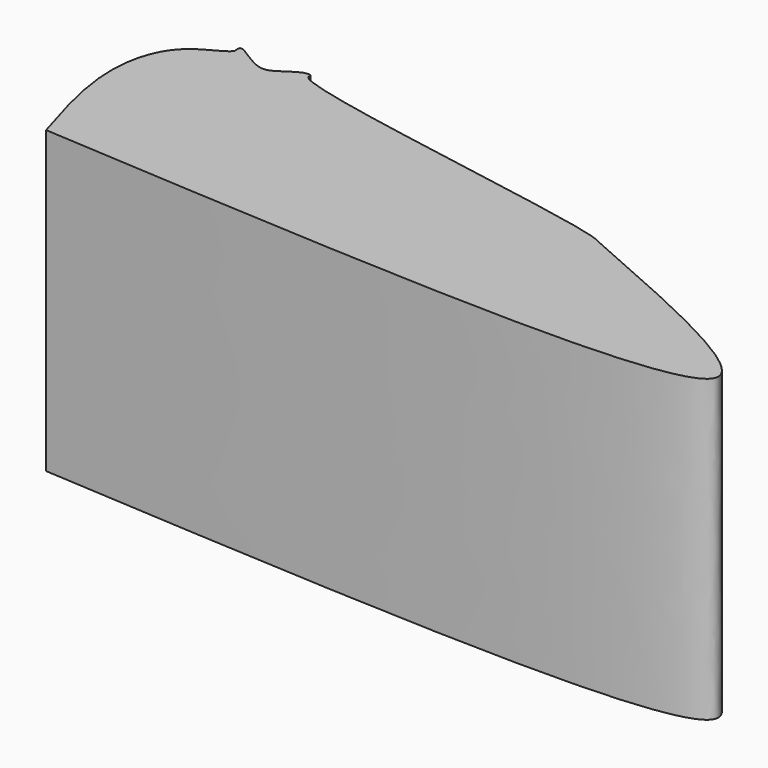
from build123d import *

# Parameters (mm, degrees)
F1_DEPTH = 25.4


with BuildPart() as f1:
    # F0 (on Top) → F1 (new body)
    with BuildSketch(Plane.XY):
        with BuildLine():
            add(Edge.make_bspline(
                [(-56.692799881, -0.0036726283), (-57.6886849621, 3.2406589588), (-59.4558836953, 9.0147803753), (-57.6335925474, 15.1716527815), (-54.2150090511, 16.1434428045), (-54.0374711329, 16.6685893238)],
                knots=[0, 0, 0, 0, 0.3642219407, 0.6481921445, 0.8580895209, 0.8580895209, 0.8580895209, 0.8580895209], degree=3))
            add(Edge.make_bspline(
                [(-18.3346489125, 10.3707137249), (-8.8863715899, 6.2547101865), (16.0703166253, -4.5953287781), (-28.8114906143, -1.7561958357), (-56.692799881, -0.0036726283)],
                knots=[0, 0, 0, 0, 0.3787092952, 1, 1, 1, 1], degree=3))
            add(Edge.make_bspline(
                [(-24.8820025145, 11.9214665673), (-22.0855730218, 11.0824777116), (-19.7342558688, 10.4620045553), (-18.3346489125, 10.3707137249)],
                knots=[0.7425998676, 0.7425998676, 0.7425998676, 0.7425998676, 0.8629450751, 0.8629450751, 0.8629450751, 0.8629450751], degree=3))
            add(Edge.make_bspline(
                [(-48.5003830651, 17.0450448134), (-48.2662958708, 17.0810595282), (-47.8080860608, 17.1514673656), (-48.6598579026, 15.8675494941), (-33.1215542234, 13.4529388682), (-24.8820025145, 11.9214665673)],
                knots=[0, 0, 0, 0, 0.0967133823, 0.1899643894, 0.7066865652, 0.7066865652, 0.7066865652, 0.7066865652], degree=3))
            add(Edge.make_bspline(
                [(-54.0643529306, 16.9809556211), (-54.0630720504, 17.0360204594), (-54.0351601992, 17.1895166337), (-53.5608966685, 17.2210881333), (-50.7884631469, 14.896841086), (-49.678037834, 16.5456728688), (-48.5003830651, 17.0450448134)],
                knots=[0.034165961, 0.034165961, 0.034165961, 0.034165961, 0.0557701507, 0.1049031527, 0.2510534482, 0.3804151484, 0.3804151484, 0.3804151484, 0.3804151484], degree=3))
            add(Edge.make_bspline(
                [(-54.0341979894, 16.678756619), (-54.0044907399, 16.7759091238), (-54.0185643259, 16.8770043639), (-54.0643529306, 16.9809556211)],
                knots=[0.8594422377, 0.8594422377, 0.8594422377, 0.8594422377, 0.8981650761, 0.8981650761, 0.8981650761, 0.8981650761], degree=3))
            add(Edge.make_bspline(
                [(-54.0374711329, 16.6685893238), (-54.0363269617, 16.6719737136), (-54.0352357619, 16.6753627606), (-54.0341979894, 16.678756619)],
                knots=[0.8580895209, 0.8580895209, 0.8580895209, 0.8580895209, 0.8594422377, 0.8594422377, 0.8594422377, 0.8594422377], degree=3))
        make_face()
        with BuildLine():
            add(Edge.make_bspline(
                [(-24.8820025145, 11.9214665673), (-22.0855730218, 11.0824777116), (-19.7342558688, 10.4620045553), (-18.3346489125, 10.3707137249)],
                knots=[0.7425998676, 0.7425998676, 0.7425998676, 0.7425998676, 0.8629450751, 0.8629450751, 0.8629450751, 0.8629450751], degree=3))
            add(Edge.make_bspline(
                [(-24.8820025145, 11.9214665673), (-21.4192914248, 11.277857994), (-18.8261043501, 10.7250289492), (-18.3346489125, 10.3707137249)],
                knots=[0.7066865652, 0.7066865652, 0.7066865652, 0.7066865652, 0.9238415357, 0.9238415357, 0.9238415357, 0.9238415357], degree=3))
        make_face()
        with BuildLine():
            add(Edge.make_bspline(
                [(-54.0341979894, 16.678756619), (-54.0502875491, 16.7863208315), (-54.0663785796, 16.8938732942), (-54.0643529306, 16.9809556211)],
                knots=[0, 0, 0, 0, 0.034165961, 0.034165961, 0.034165961, 0.034165961], degree=3))
            add(Edge.make_bspline(
                [(-54.0341979894, 16.678756619), (-54.0044907399, 16.7759091238), (-54.0185643259, 16.8770043639), (-54.0643529306, 16.9809556211)],
                knots=[0.8594422377, 0.8594422377, 0.8594422377, 0.8594422377, 0.8981650761, 0.8981650761, 0.8981650761, 0.8981650761], degree=3))
        make_face()
    extrude(amount=F1_DEPTH)


solid = f1.part
